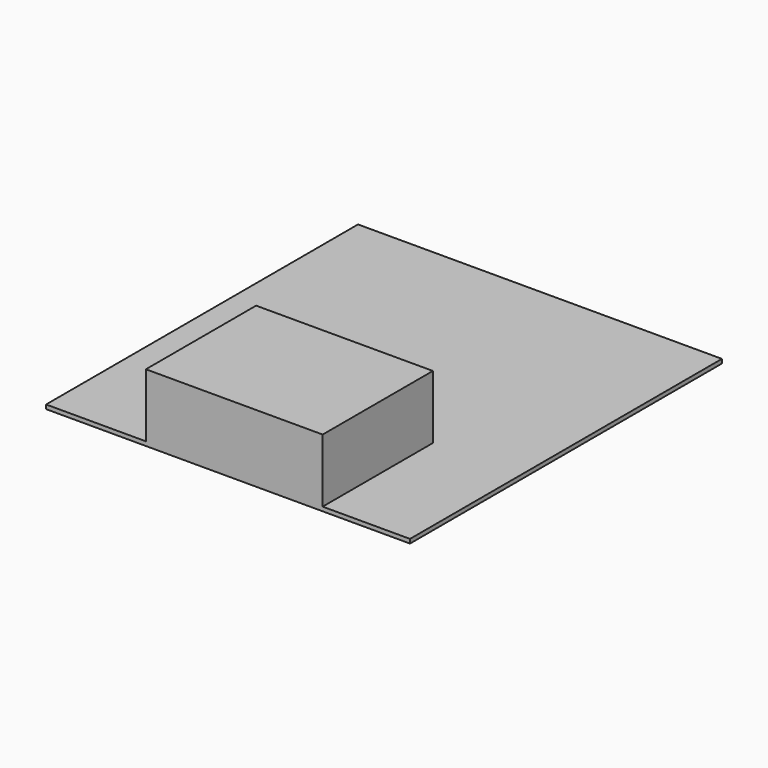
from build123d import *

# Parameters (mm, degrees)
F0_W     = 68
F0_H     = 53
F1_DEPTH = 1.5875
F2_DEPTH = 26


# Not quite as in the source:
# - a length typed as a fraction of an inch, garbled in the dataset ("3 / 203.2 mm" for 3/8 in), is restored


with BuildPart() as f1:
    # F0 (on Top) → F1 (new body)
    with BuildSketch(Plane.XY):
        Polygon((0, 150), (0, 0), (38.399413228, 0), (38.399413228, 53), (106.399413228, 53), (106.399413228, 0), (140, 0), (140, 150), align=None)
        with Locations((72.399413228, 26.5)):
            Rectangle(F0_W, F0_H)
    extrude(amount=F1_DEPTH)

    # F0 (on Top) → F2 (join)
    with BuildSketch(Plane.XY):
        with Locations((72.399413228, 26.5)):
            Rectangle(F0_W, F0_H)
    extrude(amount=F2_DEPTH)


solid = f1.part
